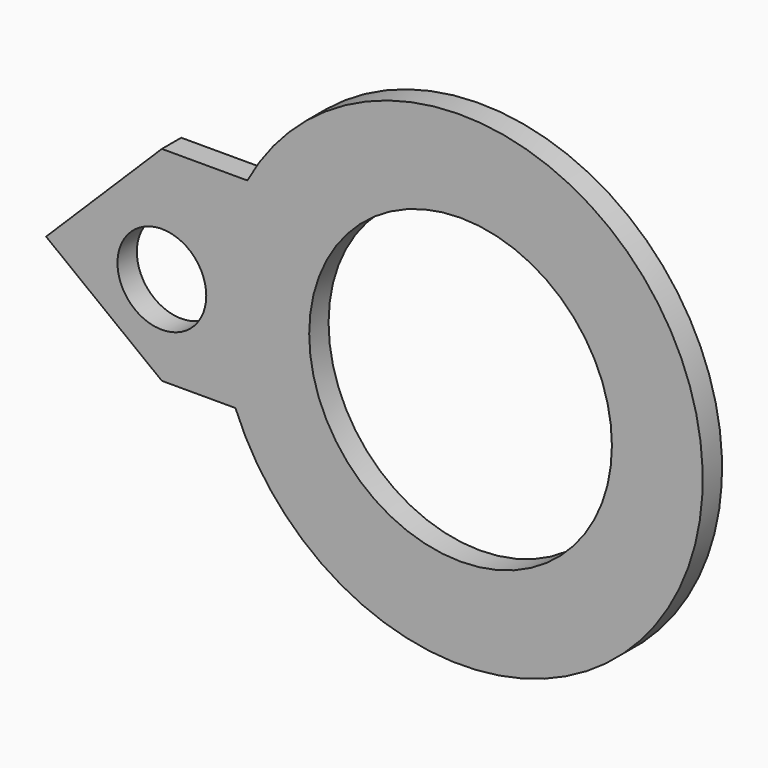
from build123d import *

# Parameters (mm, degrees)
F0_R     = 37.5
F0_R_2   = 11
F1_DEPTH = 6


# Not quite as in the source:
# - a feature names something its author has since deleted; it is built from what else it names


with BuildPart() as f1:
    # F0 (on Front) → F1 (new body)
    with BuildSketch(Plane.XZ):
        with BuildLine():
            ThreePointArc((18.2343609636, -22.1367832273), (85.2703314711, -58.932259595), (134.0014016628, 0))
            ThreePointArc((134.0014016628, 0), (88.6756766088, 58.1778794286), (21.1792131691, 28.4572732836))
            ThreePointArc((21.1792131691, 28.4572732836), (14.1027805373, 3.4864290135), (18.2343609636, -22.1367832273))
        make_face()
        with Locations((74.0014016628, 0)):
            Circle(F0_R, mode=Mode.SUBTRACT)
        with BuildLine():
            ThreePointArc((18.2343609636, -22.1367832273), (14.1027805373, 3.4864290135), (21.1792131691, 28.4572732836))
            Line((21.1792131691, 28.4572732836), (0, 28.4572732836))
            Line((0, 28.4572732836), (-28.6835413426, 0))
            Line((-28.6835413426, 0), (0, -22.1367832273))
            Line((0, -22.1367832273), (18.2343609636, -22.1367832273))
        make_face()
        Circle(F0_R_2, mode=Mode.SUBTRACT)
    extrude(amount=F1_DEPTH)


solid = f1.part
